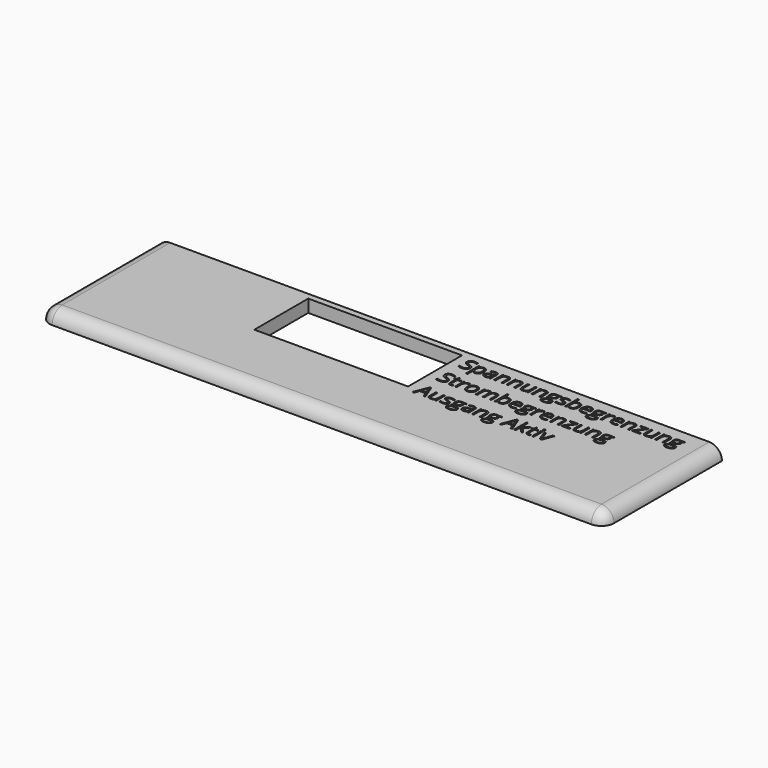
from build123d import *

# Parameters (mm, degrees)
F0_W         = 134
F0_H         = 35
F0_W_2       = 33
F0_H_2       = 7
F0_W_3       = 36.5
F0_H_3       = 16
F1_DEPTH     = 3
F2_R         = 2.99999
F3_DEPTH     = 2
F4_TEXT_SIZE = 4.8611111111
F5_DEPTH     = 1


# Not quite as in the source:
# - a fillet or chamfer is up to 0.001 mm smaller than in the source, because OpenCascade refuses the exact size
# - Text() gives the source's letters only with a copy of the font that has no kerning and outlines rounded to 1/6400 em; it was checked with that copy


with BuildPart() as f1:
    # F0 (on Top) → F1 (new body)
    with BuildSketch(Plane.XY):
        with Locations((-67, -17.5)):
            Rectangle(F0_W, F0_H)
        with Locations((-75.5, -25.5)):
            Rectangle(F0_W_2, F0_H_2, mode=Mode.SUBTRACT)
        with Locations((-78.75, -9.5)):
            Rectangle(F0_W_3, F0_H_3, mode=Mode.SUBTRACT)
        with Locations((-75.5, -25.5)):
            Rectangle(F0_W_2, F0_H_2)
    extrude(amount=F1_DEPTH)

    # F2 (radius 3 in the source; OpenCascade refuses exactly that, so slightly less here)
    f2_edges = [f1.edges().sort_by_distance(p)[0] for p in [
        (-67, -35, 3),
        (-134, -17.5, 3),
        (0, -17.5, 3),
        (-134, -35, 1.5),
        (0, -35, 1.5),
    ]]
    fillet(f2_edges, radius=F2_R)

    # F0 (on Top) → F3 (cut)
    with BuildSketch(Plane.XY):
        with Locations((-75.5, -25.5)):
            Rectangle(F0_W_2, F0_H_2)
    extrude(amount=F3_DEPTH, mode=Mode.SUBTRACT)

    # F4 (on face) → F5 (cut)
    with BuildSketch(Plane.XY.offset(3)):
        with Locations((-58.5, -5.5)):
            Text('Spannungsbegrenzung', F4_TEXT_SIZE, font='Open Sans', text_align=(TextAlign.LEFT, TextAlign.BOTTOM))
        with Locations((-58.5, -12.1111111111)):
            Text('Strombegrenzung', F4_TEXT_SIZE, font='Open Sans', text_align=(TextAlign.LEFT, TextAlign.BOTTOM))
        with Locations((-58.5, -18.7222222222)):
            Text('Ausgang Aktiv', F4_TEXT_SIZE, font='Open Sans', text_align=(TextAlign.LEFT, TextAlign.BOTTOM))
    extrude(amount=-F5_DEPTH, mode=Mode.SUBTRACT)


solid = f1.part
